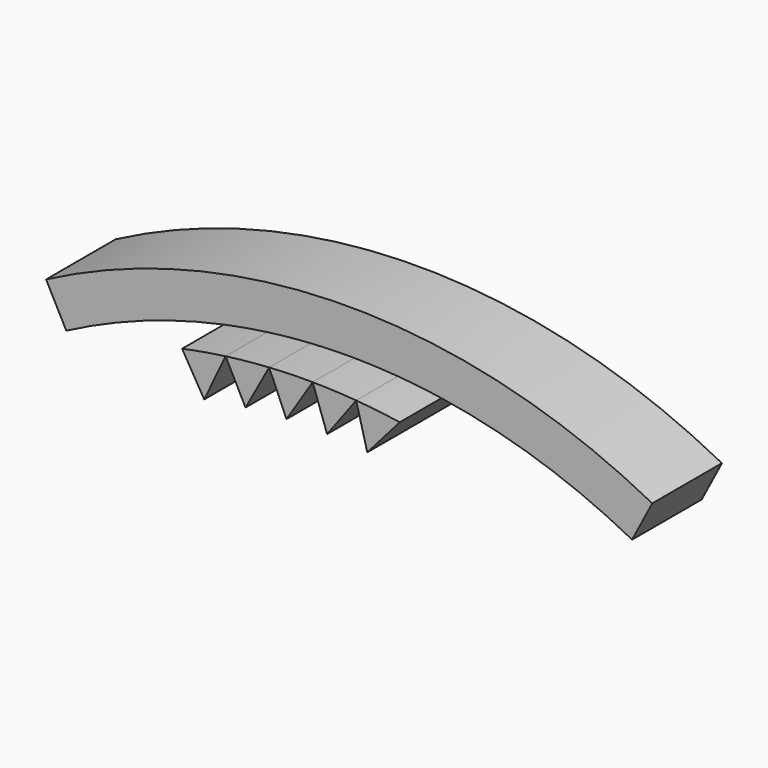
from build123d import *

# Parameters (mm, degrees)
F1_DEPTH      = 12.7
F3_DEPTH      = 7.62
F3_DEPTH_BACK = 12.7


with BuildPart() as f1:
    # F0 (on Front) → F1 (new body)
    with BuildSketch(Plane.XZ):
        with BuildLine():
            Line((-2.947556559, 5.6244480686), (0, 0))
            ThreePointArc((0, 0), (41.275, 10.16), (82.55, 0))
            Line((82.55, 0), (85.497556559, 5.6244480686))
            ThreePointArc((85.497556559, 5.6244480686), (41.275, 16.5100004524), (-2.947556559, 5.6244480686))
        make_face()
    extrude(amount=F1_DEPTH)

    # F2 (on face) → F3, piece 4 (join, two sides)
    with BuildSketch(Plane.XZ.offset(12.7)) as f3_4_sk:
        with BuildLine():
            ThreePointArc((29.3410407992, 9.35553079), (26.156112774, 8.8652546041), (22.9910407992, 8.2598979669))
            Line((22.9910407992, 8.2598979669), (26.2207533036, 2.7925899328))
            Line((26.2207533036, 2.7925899328), (29.3410407992, 9.35553079))
        make_face()
        with BuildLine():
            ThreePointArc((54.7410407992, 9.1344356868), (51.5726966653, 9.561705466), (48.3910407992, 9.8748028385))
            Line((48.3910407992, 9.8748028385), (50.0112283643, 3.7349744815))
            Line((50.0112283643, 3.7349744815), (54.7410407992, 9.1344356868))
        make_face()
    extrude(amount=F3_DEPTH)
    extrude(f3_4_sk.sketch, amount=-F3_DEPTH_BACK)


with BuildPart() as f3:
    # F2 (on face) → F3 (new body, two sides)
    with BuildSketch(Plane.XZ.offset(12.7)) as f3_sk:
        with BuildLine():
            ThreePointArc((35.6910407992, 9.9844969832), (32.5103969914, 9.7269933877), (29.3410407992, 9.35553079))
            Line((29.3410407992, 9.35553079), (32.2480694866, 3.7100295535))
            Line((32.2480694866, 3.7100295535), (35.6910407992, 9.9844969832))
        make_face()
    extrude(amount=F3_DEPTH)
    extrude(f3_sk.sketch, amount=-F3_DEPTH_BACK)


with BuildPart() as f3b:
    # F2 (on face) → F3, piece 2 (new body, two sides)
    with BuildSketch(Plane.XZ.offset(12.7)) as f3_2_sk:
        with BuildLine():
            ThreePointArc((42.0410407992, 10.1567002338), (38.8645025574, 10.1273213224), (35.6910407992, 9.9844969832))
            Line((35.6910407992, 9.9844969832), (38.2253531935, 4.1621468831))
            Line((38.2253531935, 4.1621468831), (42.0410407992, 10.1567002338))
        make_face()
    extrude(amount=F3_DEPTH)
    extrude(f3_2_sk.sketch, amount=-F3_DEPTH_BACK)


with BuildPart() as f3c:
    # F2 (on face) → F3, piece 3 (new body, two sides)
    with BuildSketch(Plane.XZ.offset(12.7)) as f3_3_sk:
        with BuildLine():
            ThreePointArc((48.3910407992, 9.8748028385), (45.2185604619, 10.0725092719), (42.0410407992, 10.1567002338))
            Line((42.0410407992, 10.1567002338), (44.1476118764, 4.1663030602))
            Line((44.1476118764, 4.1663030602), (48.3910407992, 9.8748028385))
        make_face()
    extrude(amount=F3_DEPTH)
    extrude(f3_3_sk.sketch, amount=-F3_DEPTH_BACK)


solid = Compound([f1.part, f3.part, f3b.part, f3c.part])
